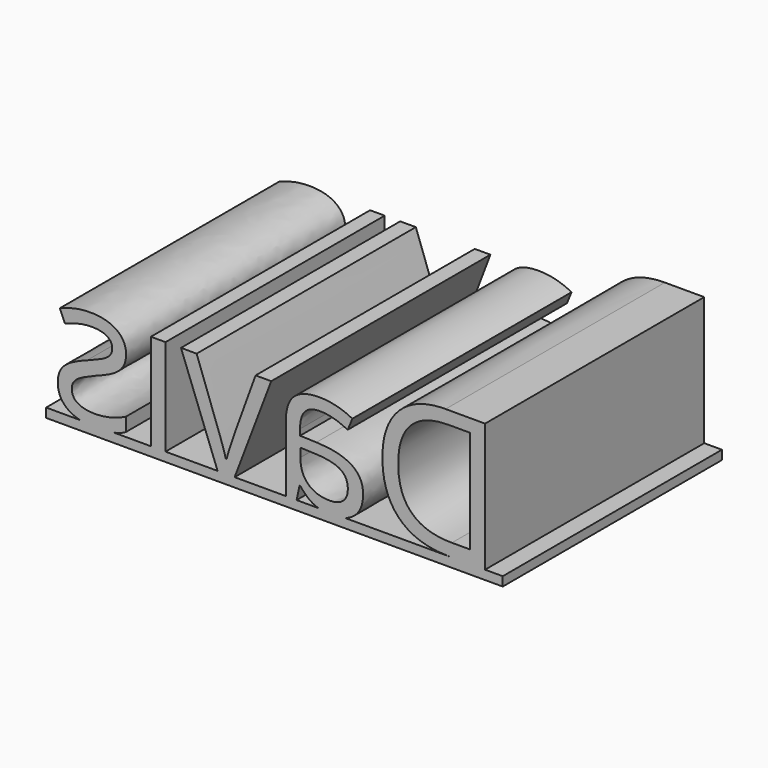
from build123d import *

# Parameters (mm, degrees)
F0_W         = 127
F0_H         = 2.54
F1_DEPTH     = 76.2
F2_TEXT_SIZE = 50.0986193294
F3_DEPTH     = 76.2
F4_W         = 7.921712473
F4_H         = 10.5424672365
F5_DEPTH     = 127


# Not quite as in the source:
# - Text() gives the source's letters only with a copy of the font that has no kerning and outlines rounded to 1/6400 em; it was checked with that copy


with BuildPart() as f1:
    # F0 (on Front) → F1 (new body)
    with BuildSketch(Plane.XZ):
        with Locations((63.5, 1.27)):
            Rectangle(F0_W, F0_H)
    extrude(amount=F1_DEPTH)

    # F2 (on face) → F3 (join)
    with BuildSketch(Plane(origin=(0, 0, 0), x_dir=(-1, 0, 0), z_dir=(0, 1, 0))):
        with Locations((-127, 2.54)):
            Text('Davis', F2_TEXT_SIZE, font='Open Sans', text_align=(TextAlign.LEFT, TextAlign.BOTTOM))
    extrude(amount=-F3_DEPTH)

    # F4 (on face) → F5 (cut)
    with BuildSketch(Plane(origin=(0, 0, 0), x_dir=(-1, 0, 0), z_dir=(0, 1, 0))):
        with Locations((-31.3993906602, 38.5790653527)):
            Rectangle(F4_W, F4_H)
    extrude(amount=-F5_DEPTH, mode=Mode.SUBTRACT)


solid = f1.part
